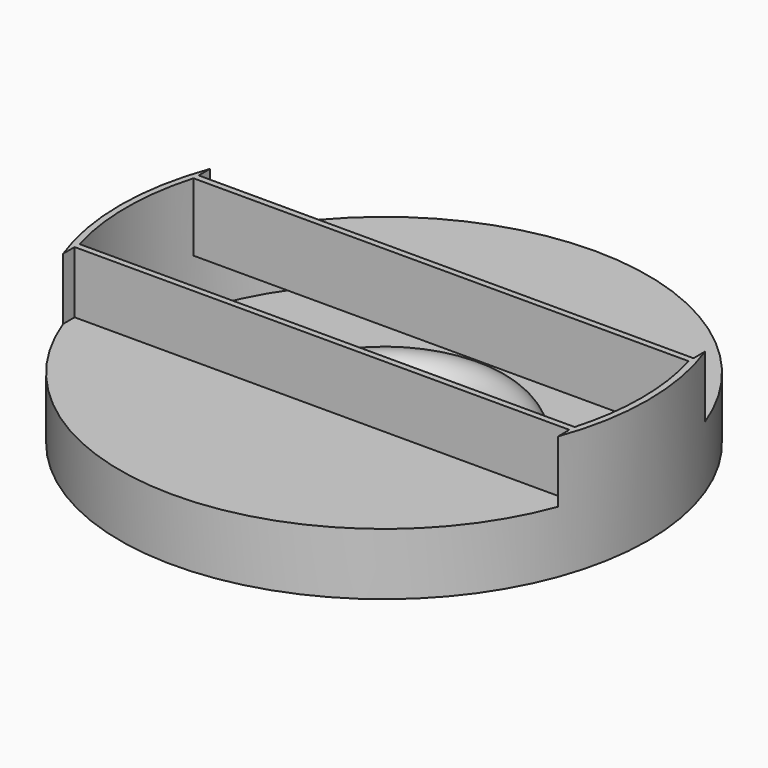
from build123d import *

# Parameters (mm, degrees)
F0_R        = 106.68
F1_DEPTH    = 50
F2_R        = 9
F4_W        = 88.5786805532
F4_H        = 25.534863025
F5_DEPTH    = 100
F6_T        = 2.54
F6_T3_DEPTH = 30.08
F6_T5_DEPTH = 10.8915489546
F6_T7_DEPTH = 205.08
F6_T9_DEPTH = 10.8915489546


# Not quite as in the source:
# - a shell that OpenCascade refuses in one call is made with other operations: the cavity is built on its own and cut out


with BuildPart() as f1:
    # F0 (on Top) → F1 (new body)
    with BuildSketch(Plane.XY):
        Circle(F0_R)
    extrude(amount=F1_DEPTH)

    # F2 (on Front) → F3 (revolve, cut)
    with BuildSketch(Plane.XZ):
        with Locations((41.004, 0)):
            Circle(F2_R)
    revolve(axis=Axis((0, 0, 20.5781124532), (0, 0, 1)), mode=Mode.SUBTRACT)

    # F4 (on Right) → F5 (cut, symmetric)
    with BuildSketch(Plane.YZ):
        with Locations((75.6345188421, 37.7674315125)):
            Rectangle(F4_W, F4_H)
        with Locations((-75.6345188421, 37.7674315125)):
            Rectangle(F4_W, F4_H)
    extrude(amount=F5_DEPTH, both=True, mode=Mode.SUBTRACT)

    # F6: shell of thickness 2.54, made by hand


with BuildPart() as f6_core1:
    # F6_t2: copy of F1
    add(f1.part)

    # the walls: a layer under each face that stays
    f6_faces = [f6_core1.faces().sort_by_distance(p)[0] for p in [
        (-106.68, 0, 25),
        (-71.12, -71.12, 0),
        (100, -34.2509530428, 37.5),
        (0, -69.0125892827, 25),
        (-100, -34.2509530428, 37.5),
        (-100, 34.2509530428, 37.5),
        (0, 69.0125892827, 25),
        (100, 34.2509530428, 37.5),
        (-41.004, 0, 9),
        (0, -31.3451785655, 37.5),
        (0, 31.3451785655, 37.5),
        (0, 0, 0),
    ]]
    thicken(f6_faces, amount=-F6_T, mode=Mode.SUBTRACT)

    # F6_s4 → F6_t3 (cut)
    with BuildSketch(Plane.XY.offset(22.46)):
        Polygon((99.9746, -31.3705785655), (102.54, -31.3451785655), (102.54, -28.8051785655), (100, -28.8051785655), align=None)
        Polygon((-99.9746, -31.3705785655), (-102.54, -31.3451785655), (-102.54, -28.8051785655), (-100, -28.8051785655), align=None)
        Polygon((-99.9746, 31.3705785655), (-102.54, 31.3451785655), (-102.54, 28.8051785655), (-100, 28.8051785655), align=None)
        Polygon((99.9746, 31.3705785655), (102.54, 31.3451785655), (102.54, 28.8051785655), (100, 28.8051785655), align=None)
    extrude(amount=F6_T3_DEPTH, mode=Mode.SUBTRACT)

    # F6_s6 → F6_t5 (cut)
    with BuildSketch(Plane.XZ.offset(28.8051785655)):
        Polygon((99.9746, 25.0254), (102.54, 25), (102.54, 22.46), (100, 22.46), align=None)
        Polygon((-99.9746, 25.0254), (-100, 22.46), (-102.54, 22.46), (-102.54, 25), align=None)
    extrude(amount=F6_T5_DEPTH, mode=Mode.SUBTRACT)

    # F6_s8 → F6_t7 (cut)
    with BuildSketch(Plane.YZ.offset(-102.54)):
        Polygon((-31.3705785655, 25.0254), (-31.3451785655, 22.46), (-28.8051785655, 22.46), (-28.8051785655, 25), align=None)
        Polygon((31.3705785655, 25.0254), (31.3451785655, 22.46), (28.8051785655, 22.46), (28.8051785655, 25), align=None)
    extrude(amount=F6_T7_DEPTH, mode=Mode.SUBTRACT)

    # F6_s10 → F6_t9 (cut)
    with BuildSketch(Plane.XZ.offset(-39.6967275201)):
        Polygon((-99.9746, 25.0254), (-102.54, 25), (-102.54, 22.46), (-100, 22.46), align=None)
        Polygon((99.9746, 25.0254), (100, 22.46), (102.54, 22.46), (102.54, 25), align=None)
    extrude(amount=F6_T9_DEPTH, mode=Mode.SUBTRACT)


with BuildPart() as f1_1:
    add(f1.part)

    # what is left inside the walls is the cavity
    f6_cavity = [f6_core1.part.solids().sort_by_distance(p)[0] for p in [
        (-52.07, 34.713333, 2.5654),
    ]]
    add(f6_cavity, mode=Mode.SUBTRACT)


solid = f1_1.part
